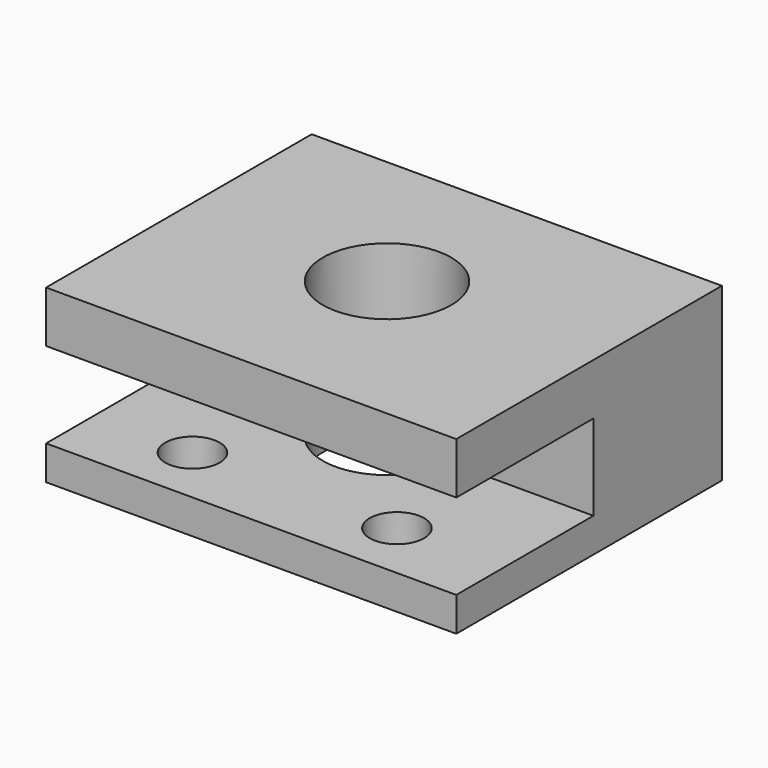
from build123d import *

# Parameters (mm, degrees)
F0_W     = 95.7474842701
F0_H     = 77.4886654093
F0_R     = 15
F1_DEPTH = 40
F2_W     = 95.7474842701
F2_H     = 20
F3_DEPTH = 40
F4_R     = 6.3464300443
F5_DEPTH = 25


# Not quite as in the source:
# - a pattern or mirror of a feature is missing from the dataset's text; its kind, count and spacing are read off the source's solid


with BuildPart() as f1:
    # F0 (on Top) → F1 (new body)
    with BuildSketch(Plane.XY):
        with Locations((0.8906734218, -2.0040220562)):
            Rectangle(F0_W, F0_H)
        Circle(F0_R, mode=Mode.SUBTRACT)
    extrude(amount=F1_DEPTH)

    # F2 (on face) → F3 (cut)
    with BuildSketch(Plane.XZ.offset(40.7483547609)):
        with Locations((0.8906734218, 17.9856412485)):
            Rectangle(F2_W, F2_H)
    extrude(amount=-F3_DEPTH, mode=Mode.SUBTRACT)

    # F4 (on face) → F5 (cut)
    with BuildSketch(Plane(origin=(0, 0, 0), x_dir=(1, 0, 0), z_dir=(0, 0, -1))):
        with Locations((23.8608885556, 26.9455648959)):
            Circle(F4_R)
    f5 = extrude(amount=-F5_DEPTH, mode=Mode.SUBTRACT)

    # F5_copies: F5 across plane
    add(f5.mirror(Plane(origin=(0, 0, 0), x_dir=(0, 0, -1), z_dir=(-1, 0, 0))), mode=Mode.SUBTRACT)


solid = f1.part
